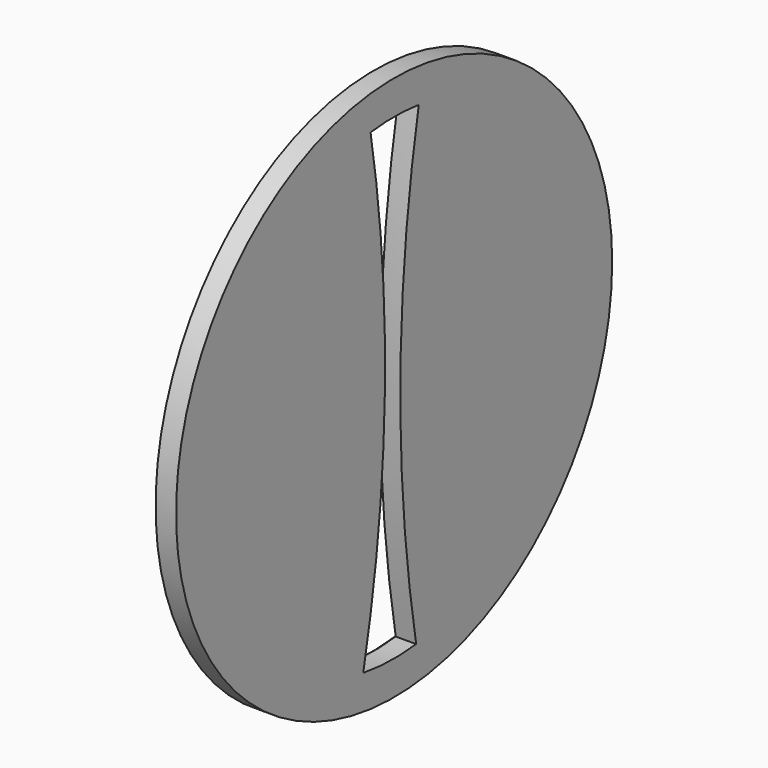
from build123d import *

# Parameters (mm, degrees)
F0_R     = 508
F1_DEPTH = 38.1
F4_D     = 889
F6_DEPTH = 38.1
F7_R     = 449.2110909422
F7_R_2   = 448.3937142921
F8_DEPTH = 5.08


with BuildPart() as f1:
    # F0 (on Right) → F1 (new body)
    with BuildSketch(Plane.YZ):
        Circle(F0_R)
    extrude(amount=F1_DEPTH)

    # F4 (through all)
    with Locations(Plane.YZ.offset(38.1)):
        with Locations((0, 0)):
            Hole(F4_D / 2)

    # F5 (on face) → F6 (join)
    with BuildSketch(Plane(origin=(0, 0, 0), x_dir=(0, -1, 0), z_dir=(-1, 0, 0))):
        with BuildLine():
            ThreePointArc((444.5, 0), (333.1536714942, 294.2598871235), (54.8987348933, 441.0967908601))
            ThreePointArc((54.8987348933, 441.0967908601), (21.5516885972, 0.4157843691), (71.8712062792, -438.6510910826))
            ThreePointArc((71.8712062792, -438.6510910826), (338.767620347, -287.7789940292), (444.5, 0))
        make_face()
        with BuildLine():
            ThreePointArc((-51.3196943653, -441.5275064707), (-14.4431317717, -0.1011743755), (-57.5001694311, 440.7652215357))
            ThreePointArc((-57.5001694311, 440.7652215357), (-444.4890945371, -3.1136534152), (-51.3196943653, -441.5275064707))
        make_face()
    extrude(amount=-F6_DEPTH)

    # F7 (on face) → F8 (join)
    with BuildSketch(Plane(origin=(0, 0, 0), x_dir=(0, -1, 0), z_dir=(-1, 0, 0))):
        Circle(F7_R)
        Circle(F7_R_2, mode=Mode.SUBTRACT)
    extrude(amount=F8_DEPTH)


solid = f1.part
